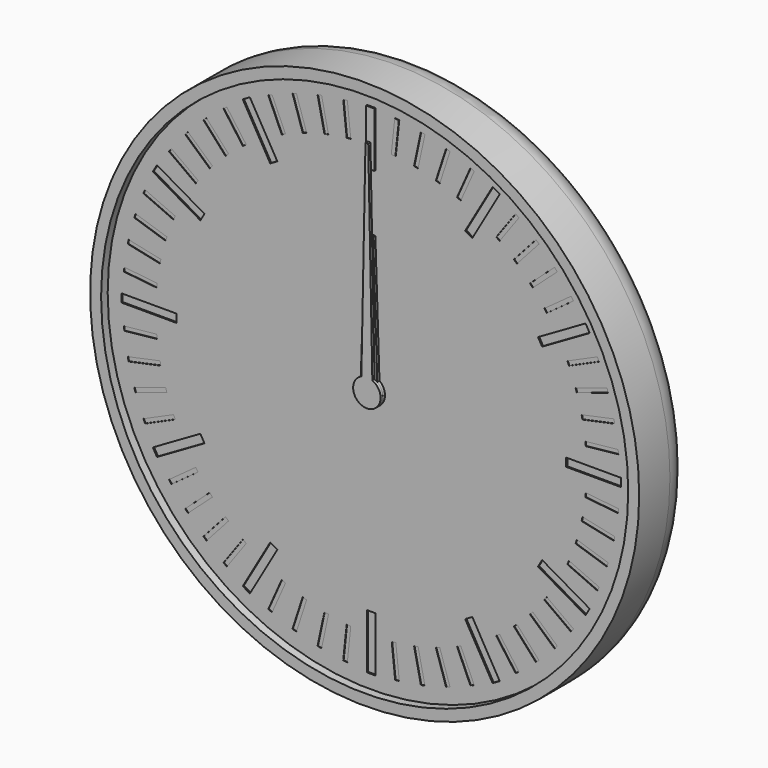
from build123d import *

# Parameters (mm, degrees)
F0_R      = 100
F1_DEPTH  = 24
F2_R      = 10
F3_T      = -4
F4_R      = 5
F4_R_2    = 3
F5_DEPTH  = 2
F6_DEPTH  = 19
F7_DEPTH  = 8
F9_DEPTH  = 4
F11_DEPTH = 4
F12_R     = 5
F12_R_2   = 3
F13_DEPTH = 2
F14_R     = 3
F15_DEPTH = 4
F17_DEPTH = 4
F18_R     = 3
F19_DEPTH = 4
F20_R     = 98
F20_R_2   = 5
F21_DEPTH = 1
F23_R     = 5
F23_R_2   = 3
F24_DEPTH = 4
F25_W     = 3
F25_H     = 20
F25_W_2   = 20
F25_H_2   = 3
F26_DEPTH = 0.5
F27_W     = 1.5
F27_H     = 12
F27_W_2   = 12
F27_H_2   = 1.5
F28_DEPTH = 0.2
F29_DEPTH = 1
F30_DEPTH = 0.4
F31_R     = 5
F31_R_2   = 3
F32_DEPTH = 5
F33_R     = 3
F34_DEPTH = 1
F36_DEPTH = 1


with BuildPart() as f1:
    # F0 (on Front) → F1 (new body)
    with BuildSketch(Plane.XZ):
        Circle(F0_R)
    extrude(amount=F1_DEPTH)

    # F2
    f2_edges = [f1.edges().sort_by_distance(p)[0] for p in [
        (-100, 0, 0),
    ]]
    fillet(f2_edges, radius=F2_R)

    # F3
    f3_openings = [f1.faces().sort_by_distance(p)[0] for p in [
        (0, -24, 0),
    ]]
    offset(amount=F3_T, openings=f3_openings)

    # F4 (on face) → F5 (join)
    with BuildSketch(Plane.XZ.offset(4)):
        Circle(F4_R)
        Circle(F4_R_2, mode=Mode.SUBTRACT)
        with Locations((40, 0)):
            Circle(F4_R)
        with Locations((40, 0)):
            Circle(F4_R_2, mode=Mode.SUBTRACT)
    extrude(amount=F5_DEPTH)


with BuildPart() as f6:
    # F6 (new): a face of the model
    f6_faces = [f1.part.faces().sort_by_distance(p)[0] for p in [
        (0, -4, 0),
    ]]
    extrude(f6_faces, amount=F6_DEPTH)

    # F8 (on face) → F9 (join)
    with BuildSketch(Plane.XZ.offset(6)):
        with BuildLine():
            ThreePointArc((9.2729637667, -1.3794085621), (9.3494561423, -0.6915886375), (9.375, 0))
            ThreePointArc((9.375, 0), (9.3494561423, 0.6915886375), (9.2729637667, 1.3794085621))
            ThreePointArc((9.2729637667, 1.3794085621), (8.9161548403, 2.8970343223), (8.3127812852, 4.3345463782))
            ThreePointArc((8.3127812852, 4.3345463782), (7.5845343223, 5.5104867402), (6.6911892658, 6.566476316))
            ThreePointArc((6.6911892658, 6.566476316), (5.5104867402, 7.5845343223), (4.1773988938, 8.3928519278))
            ThreePointArc((4.1773988938, 8.3928519278), (2.8970343223, 8.9161548403), (1.5536078905, 9.2453733036))
            ThreePointArc((1.5536078905, 9.2453733036), (0, 9.375), (-1.5536078905, 9.2453733036))
            ThreePointArc((-1.5536078905, 9.2453733036), (-2.8970343223, 8.9161548403), (-4.1773988938, 8.3928519278))
            ThreePointArc((-4.1773988938, 8.3928519278), (-5.5104867402, 7.5845343223), (-6.6911892658, 6.566476316))
            ThreePointArc((-6.6911892658, 6.566476316), (-7.5845343223, 5.5104867402), (-8.3127812852, 4.3345463782))
            ThreePointArc((-8.3127812852, 4.3345463782), (-8.9161548403, 2.8970343223), (-9.2729637667, 1.3794085621))
            ThreePointArc((-9.2729637667, 1.3794085621), (-9.375, 0), (-9.2729637667, -1.3794085621))
            ThreePointArc((-9.2729637667, -1.3794085621), (-8.9161548403, -2.8970343223), (-8.3127812852, -4.3345463782))
            ThreePointArc((-8.3127812852, -4.3345463782), (-7.5845343223, -5.5104867402), (-6.6911892658, -6.566476316))
            ThreePointArc((-6.6911892658, -6.566476316), (-5.5104867402, -7.5845343223), (-4.1773988938, -8.3928519278))
            ThreePointArc((-4.1773988938, -8.3928519278), (-2.8970343223, -8.9161548403), (-1.5536078905, -9.2453733036))
            ThreePointArc((-1.5536078905, -9.2453733036), (0, -9.375), (1.5536078905, -9.2453733036))
            ThreePointArc((1.5536078905, -9.2453733036), (2.8970343223, -8.9161548403), (4.1773988938, -8.3928519278))
            ThreePointArc((4.1773988938, -8.3928519278), (5.5104867402, -7.5845343223), (6.6911892658, -6.566476316))
            ThreePointArc((6.6911892658, -6.566476316), (7.5845343223, -5.5104867402), (8.3127812852, -4.3345463782))
            ThreePointArc((8.3127812852, -4.3345463782), (8.9161548403, -2.8970343223), (9.2729637667, -1.3794085621))
        make_face()
        with BuildLine():
            ThreePointArc((8.3127812852, 4.3345463782), (8.9161548403, 2.8970343223), (9.2729637667, 1.3794085621))
            Line((9.2729637667, 1.3794085621), (11.1823199426, 2.3946312492))
            Line((11.1823199426, 2.3946312492), (10.8182678729, 3.515068311))
            Line((10.8182678729, 3.515068311), (10.4542158031, 4.6355053728))
            Line((10.4542158031, 4.6355053728), (8.3127812852, 4.3345463782))
        make_face()
        with BuildLine():
            Line((11.1823199426, -2.3946312492), (9.2729637667, -1.3794085621))
            ThreePointArc((9.2729637667, -1.3794085621), (8.9161548403, -2.8970343223), (8.3127812852, -4.3345463782))
            Line((8.3127812852, -4.3345463782), (10.4542158031, -4.6355053728))
            Line((10.4542158031, -4.6355053728), (10.8182678729, -3.515068311))
            Line((10.8182678729, -3.515068311), (11.1823199426, -2.3946312492))
        make_face()
        with BuildLine():
            ThreePointArc((4.1773988938, 8.3928519278), (5.5104867402, 7.5845343223), (6.6911892658, 6.566476316))
            Line((6.6911892658, 6.566476316), (7.6391579371, 8.5101001246))
            Line((7.6391579371, 8.5101001246), (6.6860572448, 9.202568311))
            Line((6.6860572448, 9.202568311), (5.7329565525, 9.8950364974))
            Line((5.7329565525, 9.8950364974), (4.1773988938, 8.3928519278))
        make_face()
        with BuildLine():
            Line((7.6391579371, -8.5101001246), (6.6911892658, -6.566476316))
            ThreePointArc((6.6911892658, -6.566476316), (5.5104867402, -7.5845343223), (4.1773988938, -8.3928519278))
            Line((4.1773988938, -8.3928519278), (5.7329565525, -9.8950364974))
            Line((5.7329565525, -9.8950364974), (6.6860572448, -9.202568311))
            Line((6.6860572448, -9.202568311), (7.6391579371, -8.5101001246))
        make_face()
        with BuildLine():
            ThreePointArc((-1.5536078905, 9.2453733036), (0, 9.375), (1.5536078905, 9.2453733036))
            Line((1.5536078905, 9.2453733036), (1.1780972451, 11.375))
            Line((1.1780972451, 11.375), (0, 11.375))
            Line((0, 11.375), (-1.1780972451, 11.375))
            Line((-1.1780972451, 11.375), (-1.5536078905, 9.2453733036))
        make_face()
        with BuildLine():
            Line((1.1780972451, -11.375), (1.5536078905, -9.2453733036))
            ThreePointArc((1.5536078905, -9.2453733036), (0, -9.375), (-1.5536078905, -9.2453733036))
            Line((-1.5536078905, -9.2453733036), (-1.1780972451, -11.375))
            Line((-1.1780972451, -11.375), (0, -11.375))
            Line((0, -11.375), (1.1780972451, -11.375))
        make_face()
        with BuildLine():
            ThreePointArc((-6.6911892658, 6.566476316), (-5.5104867402, 7.5845343223), (-4.1773988938, 8.3928519278))
            Line((-4.1773988938, 8.3928519278), (-5.7329565525, 9.8950364974))
            Line((-5.7329565525, 9.8950364974), (-6.6860572448, 9.202568311))
            Line((-6.6860572448, 9.202568311), (-7.6391579371, 8.5101001246))
            Line((-7.6391579371, 8.5101001246), (-6.6911892658, 6.566476316))
        make_face()
        with BuildLine():
            Line((-5.7329565525, -9.8950364974), (-4.1773988938, -8.3928519278))
            ThreePointArc((-4.1773988938, -8.3928519278), (-5.5104867402, -7.5845343223), (-6.6911892658, -6.566476316))
            Line((-6.6911892658, -6.566476316), (-7.6391579371, -8.5101001246))
            Line((-7.6391579371, -8.5101001246), (-6.6860572448, -9.202568311))
            Line((-6.6860572448, -9.202568311), (-5.7329565525, -9.8950364974))
        make_face()
        with BuildLine():
            ThreePointArc((-9.2729637667, 1.3794085621), (-8.9161548403, 2.8970343223), (-8.3127812852, 4.3345463782))
            Line((-8.3127812852, 4.3345463782), (-10.4542158031, 4.6355053728))
            Line((-10.4542158031, 4.6355053728), (-10.8182678729, 3.515068311))
            Line((-10.8182678729, 3.515068311), (-11.1823199426, 2.3946312492))
            Line((-11.1823199426, 2.3946312492), (-9.2729637667, 1.3794085621))
        make_face()
        with BuildLine():
            Line((-10.4542158031, -4.6355053728), (-8.3127812852, -4.3345463782))
            ThreePointArc((-8.3127812852, -4.3345463782), (-8.9161548403, -2.8970343223), (-9.2729637667, -1.3794085621))
            Line((-9.2729637667, -1.3794085621), (-11.1823199426, -2.3946312492))
            Line((-11.1823199426, -2.3946312492), (-10.8182678729, -3.515068311))
            Line((-10.8182678729, -3.515068311), (-10.4542158031, -4.6355053728))
        make_face()
    extrude(amount=F9_DEPTH)

    # F35 (on face) → F36 (join)
    with BuildSketch(Plane.XZ.offset(23)):
        with BuildLine():
            ThreePointArc((-2, 4.582575695), (-2.7386127875, -4.1833001327), (5, 0))
            ThreePointArc((5, 0), (4.1833001327, 2.7386127875), (2, 4.582575695))
            ThreePointArc((2, 4.582575695), (0, 5), (-2, 4.582575695))
        make_face()
        with BuildLine():
            ThreePointArc((-2, 4.582575695), (0, 5), (2, 4.582575695))
            Line((2, 4.582575695), (0.5, 80))
            Line((0.5, 80), (0, 80))
            Line((0, 80), (-0.5, 80))
            Line((-0.5, 80), (-2, 4.582575695))
        make_face()
    extrude(amount=-F36_DEPTH)


with BuildPart() as f7:
    # F7 (new): a face of the model
    f7_faces = [f1.part.faces().sort_by_distance(p)[0] for p in [
        (40, -4, 0),
    ]]
    extrude(f7_faces, amount=F7_DEPTH)

    # F10 (on face) → F11 (join)
    with BuildSketch(Plane.XZ.offset(6)):
        with BuildLine():
            ThreePointArc((68.0829066802, -1.5381733945), (68.1144747006, -0.7693746225), (68.125, 0))
            ThreePointArc((68.125, 0), (68.1144747006, 0.7693746225), (68.0829066802, 1.5381733945))
            ThreePointArc((68.0829066802, 1.5381733945), (67.9709283072, 2.9398630294), (67.7890320221, 4.3342039956))
            ThreePointArc((67.7890320221, 4.3342039956), (67.5104012706, 5.8475163042), (67.1494235596, 7.3433252263))
            ThreePointArc((67.1494235596, 7.3433252263), (66.7484645208, 8.6911029668), (66.280643318, 10.0171558733))
            ThreePointArc((66.280643318, 10.0171558733), (65.6934659962, 11.4394680865), (65.0293803521, 12.8275385085))
            ThreePointArc((65.0293803521, 12.8275385085), (64.3569644814, 14.0625), (63.6236643925, 15.2623099717))
            ThreePointArc((63.6236643925, 15.2623099717), (62.7536029668, 16.5314602207), (61.815433119, 17.7511268046))
            ThreePointArc((61.815433119, 17.7511268046), (60.9009482166, 18.8192983038), (59.934217974, 19.8404278876))
            ThreePointArc((59.934217974, 19.8404278876), (58.8192983038, 20.9009482166), (57.6480467764, 21.8989056799))
            ThreePointArc((57.6480467764, 21.8989056799), (56.5314602207, 22.7536029668), (55.3735505752, 23.5514238999))
            ThreePointArc((55.3735505752, 23.5514238999), (54.0625, 24.3569644814), (52.709356105, 25.0895972944))
            ThreePointArc((52.709356105, 25.0895972944), (51.4394680865, 25.6934659962), (50.1409852457, 26.2331096755))
            ThreePointArc((50.1409852457, 26.2331096755), (48.6911029668, 26.7484645208), (47.2152055856, 27.1837531139))
            ThreePointArc((47.2152055856, 27.1837531139), (45.8475163042, 27.5104012706), (44.4652101991, 27.7682826779))
            ThreePointArc((44.4652101991, 27.7682826779), (42.9398630294, 27.9709283072), (41.4057159597, 28.0898484802))
            ThreePointArc((41.4057159597, 28.0898484802), (40, 28.125), (38.5942840403, 28.0898484802))
            ThreePointArc((38.5942840403, 28.0898484802), (37.0601369706, 27.9709283072), (35.5347898009, 27.7682826779))
            ThreePointArc((35.5347898009, 27.7682826779), (34.1524836958, 27.5104012706), (32.7847944144, 27.1837531139))
            ThreePointArc((32.7847944144, 27.1837531139), (31.3088970332, 26.7484645208), (29.8590147543, 26.2331096755))
            ThreePointArc((29.8590147543, 26.2331096755), (28.5605319135, 25.6934659962), (27.290643895, 25.0895972944))
            ThreePointArc((27.290643895, 25.0895972944), (25.9375, 24.3569644814), (24.6264494248, 23.5514238999))
            ThreePointArc((24.6264494248, 23.5514238999), (23.4685397793, 22.7536029668), (22.3519532236, 21.8989056799))
            ThreePointArc((22.3519532236, 21.8989056799), (21.1807016962, 20.9009482166), (20.065782026, 19.8404278876))
            ThreePointArc((20.065782026, 19.8404278876), (19.0990517834, 18.8192983038), (18.184566881, 17.7511268046))
            ThreePointArc((18.184566881, 17.7511268046), (17.2463970332, 16.5314602207), (16.3763356075, 15.2623099717))
            ThreePointArc((16.3763356075, 15.2623099717), (15.6430355186, 14.0625), (14.9706196479, 12.8275385085))
            ThreePointArc((14.9706196479, 12.8275385085), (14.3065340038, 11.4394680865), (13.719356682, 10.0171558733))
            ThreePointArc((13.719356682, 10.0171558733), (13.2515354792, 8.6911029668), (12.8505764404, 7.3433252263))
            ThreePointArc((12.8505764404, 7.3433252263), (12.4895987294, 5.8475163042), (12.2109679779, 4.3342039956))
            ThreePointArc((12.2109679779, 4.3342039956), (12.0290716928, 2.9398630294), (11.9170933198, 1.5381733945))
            ThreePointArc((11.9170933198, 1.5381733945), (11.875, 0), (11.9170933198, -1.5381733945))
            ThreePointArc((11.9170933198, -1.5381733945), (12.0290716928, -2.9398630294), (12.2109679779, -4.3342039956))
            ThreePointArc((12.2109679779, -4.3342039956), (12.4895987294, -5.8475163042), (12.8505764404, -7.3433252263))
            ThreePointArc((12.8505764404, -7.3433252263), (13.2515354792, -8.6911029668), (13.719356682, -10.0171558733))
            ThreePointArc((13.719356682, -10.0171558733), (14.3065340038, -11.4394680865), (14.9706196479, -12.8275385085))
            ThreePointArc((14.9706196479, -12.8275385085), (15.6430355186, -14.0625), (16.3763356075, -15.2623099717))
            ThreePointArc((16.3763356075, -15.2623099717), (17.2463970332, -16.5314602207), (18.184566881, -17.7511268046))
            ThreePointArc((18.184566881, -17.7511268046), (19.0990517834, -18.8192983038), (20.065782026, -19.8404278876))
            ThreePointArc((20.065782026, -19.8404278876), (21.1807016962, -20.9009482166), (22.3519532236, -21.8989056799))
            ThreePointArc((22.3519532236, -21.8989056799), (23.4685397793, -22.7536029668), (24.6264494248, -23.5514238999))
            ThreePointArc((24.6264494248, -23.5514238999), (25.9375, -24.3569644814), (27.290643895, -25.0895972944))
            ThreePointArc((27.290643895, -25.0895972944), (28.5605319135, -25.6934659962), (29.8590147543, -26.2331096755))
            ThreePointArc((29.8590147543, -26.2331096755), (31.3088970332, -26.7484645208), (32.7847944144, -27.1837531139))
            ThreePointArc((32.7847944144, -27.1837531139), (34.1524836958, -27.5104012706), (35.5347898009, -27.7682826779))
            ThreePointArc((35.5347898009, -27.7682826779), (37.0601369706, -27.9709283072), (38.5942840403, -28.0898484802))
            ThreePointArc((38.5942840403, -28.0898484802), (40, -28.125), (41.4057159597, -28.0898484802))
            ThreePointArc((41.4057159597, -28.0898484802), (42.9398630294, -27.9709283072), (44.4652101991, -27.7682826779))
            ThreePointArc((44.4652101991, -27.7682826779), (45.8475163042, -27.5104012706), (47.2152055856, -27.1837531139))
            ThreePointArc((47.2152055856, -27.1837531139), (48.6911029668, -26.7484645208), (50.1409852457, -26.2331096755))
            ThreePointArc((50.1409852457, -26.2331096755), (51.4394680865, -25.6934659962), (52.709356105, -25.0895972944))
            ThreePointArc((52.709356105, -25.0895972944), (54.0625, -24.3569644814), (55.3735505752, -23.5514238999))
            ThreePointArc((55.3735505752, -23.5514238999), (56.5314602207, -22.7536029668), (57.6480467764, -21.8989056799))
            ThreePointArc((57.6480467764, -21.8989056799), (58.8192983038, -20.9009482166), (59.934217974, -19.8404278876))
            ThreePointArc((59.934217974, -19.8404278876), (60.9009482166, -18.8192983038), (61.815433119, -17.7511268046))
            ThreePointArc((61.815433119, -17.7511268046), (62.7536029668, -16.5314602207), (63.6236643925, -15.2623099717))
            ThreePointArc((63.6236643925, -15.2623099717), (64.3569644814, -14.0625), (65.0293803521, -12.8275385085))
            ThreePointArc((65.0293803521, -12.8275385085), (65.6934659962, -11.4394680865), (66.280643318, -10.0171558733))
            ThreePointArc((66.280643318, -10.0171558733), (66.7484645208, -8.6911029668), (67.1494235596, -7.3433252263))
            ThreePointArc((67.1494235596, -7.3433252263), (67.5104012706, -5.8475163042), (67.7890320221, -4.3342039956))
            ThreePointArc((67.7890320221, -4.3342039956), (67.9709283072, -2.9398630294), (68.0829066802, -1.5381733945))
        make_face()
        with BuildLine():
            ThreePointArc((68.0829066802, 1.5381733945), (68.1144747006, 0.7693746225), (68.125, 0))
            ThreePointArc((68.125, 0), (68.1144747006, -0.7693746225), (68.0829066802, -1.5381733945))
            Line((68.0829066802, -1.5381733945), (70.125, -1.1780972451))
            Line((70.125, -1.1780972451), (70.125, 0))
            Line((70.125, 0), (70.125, 1.1780972451))
            Line((70.125, 1.1780972451), (68.0829066802, 1.5381733945))
        make_face()
        with BuildLine():
            ThreePointArc((67.1494235596, 7.3433252263), (67.5104012706, 5.8475163042), (67.7890320221, 4.3342039956))
            Line((67.7890320221, 4.3342039956), (69.7116366623, 5.1109866922))
            Line((69.7116366623, 5.1109866922), (69.4666964721, 6.2633396859))
            Line((69.4666964721, 6.2633396859), (69.2217562819, 7.4156926796))
            Line((69.2217562819, 7.4156926796), (67.1494235596, 7.3433252263))
        make_face()
        with BuildLine():
            Line((69.7116366623, -5.1109866922), (67.7890320221, -4.3342039956))
            ThreePointArc((67.7890320221, -4.3342039956), (67.5104012706, -5.8475163042), (67.1494235596, -7.3433252263))
            Line((67.1494235596, -7.3433252263), (69.2217562819, -7.4156926796))
            Line((69.2217562819, -7.4156926796), (69.4666964721, -6.2633396859))
            Line((69.4666964721, -6.2633396859), (69.7116366623, -5.1109866922))
        make_face()
        with BuildLine():
            ThreePointArc((65.0293803521, 12.8275385085), (65.6934659962, 11.4394680865), (66.280643318, 10.0171558733))
            Line((66.280643318, 10.0171558733), (67.9997322302, 11.1766959857))
            Line((67.9997322302, 11.1766959857), (67.5205569115, 12.2529413727))
            Line((67.5205569115, 12.2529413727), (67.0413815928, 13.3291867596))
            Line((67.0413815928, 13.3291867596), (65.0293803521, 12.8275385085))
        make_face()
        with BuildLine():
            Line((67.9997322302, -11.1766959857), (66.280643318, -10.0171558733))
            ThreePointArc((66.280643318, -10.0171558733), (65.6934659962, -11.4394680865), (65.0293803521, -12.8275385085))
            Line((65.0293803521, -12.8275385085), (67.0413815928, -13.3291867596))
            Line((67.0413815928, -13.3291867596), (67.5205569115, -12.2529413727))
            Line((67.5205569115, -12.2529413727), (67.9997322302, -11.1766959857))
        make_face()
        with BuildLine():
            ThreePointArc((61.815433119, 17.7511268046), (62.7536029668, 16.5314602207), (63.6236643925, 15.2623099717))
            Line((63.6236643925, 15.2623099717), (65.064105142, 16.753930033))
            Line((65.064105142, 16.753930033), (64.3716369555, 17.7070307253))
            Line((64.3716369555, 17.7070307253), (63.6791687691, 18.6601314176))
            Line((63.6791687691, 18.6601314176), (61.815433119, 17.7511268046))
        make_face()
        with BuildLine():
            Line((65.064105142, -16.753930033), (63.6236643925, -15.2623099717))
            ThreePointArc((63.6236643925, -15.2623099717), (62.7536029668, -16.5314602207), (61.815433119, -17.7511268046))
            Line((61.815433119, -17.7511268046), (63.6791687691, -18.6601314176))
            Line((63.6791687691, -18.6601314176), (64.3716369555, -17.7070307253))
            Line((64.3716369555, -17.7070307253), (65.064105142, -16.753930033))
        make_face()
        with BuildLine():
            ThreePointArc((57.6480467764, 21.8989056799), (58.8192983038, 20.9009482166), (59.934217974, 19.8404278876))
            Line((59.934217974, 19.8404278876), (61.0330563882, 21.5989369435))
            Line((61.0330563882, 21.5989369435), (60.1575595166, 22.3872378675))
            Line((60.1575595166, 22.3872378675), (59.282062645, 23.1755387915))
            Line((59.282062645, 23.1755387915), (57.6480467764, 21.8989056799))
        make_face()
        with BuildLine():
            Line((61.0330563882, -21.5989369435), (59.934217974, -19.8404278876))
            ThreePointArc((59.934217974, -19.8404278876), (58.8192983038, -20.9009482166), (57.6480467764, -21.8989056799))
            Line((57.6480467764, -21.8989056799), (59.282062645, -23.1755387915))
            Line((59.282062645, -23.1755387915), (60.1575595166, -22.3872378675))
            Line((60.1575595166, -22.3872378675), (61.0330563882, -21.5989369435))
        make_face()
        with BuildLine():
            ThreePointArc((52.709356105, 25.0895972944), (54.0625, 24.3569644814), (55.3735505752, 23.5514238999))
            Line((55.3735505752, 23.5514238999), (56.0827621424, 25.4999666665))
            Line((56.0827621424, 25.4999666665), (55.0625, 26.089015289))
            Line((55.0625, 26.089015289), (54.0422378576, 26.6780639116))
            Line((54.0422378576, 26.6780639116), (52.709356105, 25.0895972944))
        make_face()
        with BuildLine():
            Line((56.0827621424, -25.4999666665), (55.3735505752, -23.5514238999))
            ThreePointArc((55.3735505752, -23.5514238999), (54.0625, -24.3569644814), (52.709356105, -25.0895972944))
            Line((52.709356105, -25.0895972944), (54.0422378576, -26.6780639116))
            Line((54.0422378576, -26.6780639116), (55.0625, -26.089015289))
            Line((55.0625, -26.089015289), (56.0827621424, -25.4999666665))
        make_face()
        with BuildLine():
            ThreePointArc((47.2152055856, 27.1837531139), (48.6911029668, 26.7484645208), (50.1409852457, 26.2331096755))
            Line((50.1409852457, 26.2331096755), (50.4295740173, 28.2865254836))
            Line((50.4295740173, 28.2865254836), (49.3091369555, 28.6505775534))
            Line((49.3091369555, 28.6505775534), (48.1886998938, 29.0146296232))
            Line((48.1886998938, 29.0146296232), (47.2152055856, 27.1837531139))
        make_face()
        with BuildLine():
            Line((50.4295740173, -28.2865254836), (50.1409852457, -26.2331096755))
            ThreePointArc((50.1409852457, -26.2331096755), (48.6911029668, -26.7484645208), (47.2152055856, -27.1837531139))
            Line((47.2152055856, -27.1837531139), (48.1886998938, -29.0146296232))
            Line((48.1886998938, -29.0146296232), (49.3091369555, -28.6505775534))
            Line((49.3091369555, -28.6505775534), (50.4295740173, -28.2865254836))
        make_face()
        with BuildLine():
            ThreePointArc((41.4057159597, 28.0898484802), (42.9398630294, 27.9709283072), (44.4652101991, 27.7682826779))
            Line((44.4652101991, 27.7682826779), (44.3205634611, 29.8368274034))
            Line((44.3205634611, 29.8368274034), (43.1489199559, 29.959972098))
            Line((43.1489199559, 29.959972098), (41.9772764508, 30.0831167926))
            Line((41.9772764508, 30.0831167926), (41.4057159597, 28.0898484802))
        make_face()
        with BuildLine():
            Line((44.3205634611, -29.8368274034), (44.4652101991, -27.7682826779))
            ThreePointArc((44.4652101991, -27.7682826779), (42.9398630294, -27.9709283072), (41.4057159597, -28.0898484802))
            Line((41.4057159597, -28.0898484802), (41.9772764508, -30.0831167926))
            Line((41.9772764508, -30.0831167926), (43.1489199559, -29.959972098))
            Line((43.1489199559, -29.959972098), (44.3205634611, -29.8368274034))
        make_face()
        with BuildLine():
            ThreePointArc((35.5347898009, 27.7682826779), (37.0601369706, 27.9709283072), (38.5942840403, 28.0898484802))
            Line((38.5942840403, 28.0898484802), (38.0227235492, 30.0831167926))
            Line((38.0227235492, 30.0831167926), (36.8510800441, 29.959972098))
            Line((36.8510800441, 29.959972098), (35.6794365389, 29.8368274034))
            Line((35.6794365389, 29.8368274034), (35.5347898009, 27.7682826779))
        make_face()
        with BuildLine():
            Line((38.0227235492, -30.0831167926), (38.5942840403, -28.0898484802))
            ThreePointArc((38.5942840403, -28.0898484802), (37.0601369706, -27.9709283072), (35.5347898009, -27.7682826779))
            Line((35.5347898009, -27.7682826779), (35.6794365389, -29.8368274034))
            Line((35.6794365389, -29.8368274034), (36.8510800441, -29.959972098))
            Line((36.8510800441, -29.959972098), (38.0227235492, -30.0831167926))
        make_face()
        with BuildLine():
            ThreePointArc((29.8590147543, 26.2331096755), (31.3088970332, 26.7484645208), (32.7847944144, 27.1837531139))
            Line((32.7847944144, 27.1837531139), (31.8113001062, 29.0146296232))
            Line((31.8113001062, 29.0146296232), (30.6908630445, 28.6505775534))
            Line((30.6908630445, 28.6505775534), (29.5704259827, 28.2865254836))
            Line((29.5704259827, 28.2865254836), (29.8590147543, 26.2331096755))
        make_face()
        with BuildLine():
            Line((31.8113001062, -29.0146296232), (32.7847944144, -27.1837531139))
            ThreePointArc((32.7847944144, -27.1837531139), (31.3088970332, -26.7484645208), (29.8590147543, -26.2331096755))
            Line((29.8590147543, -26.2331096755), (29.5704259827, -28.2865254836))
            Line((29.5704259827, -28.2865254836), (30.6908630445, -28.6505775534))
            Line((30.6908630445, -28.6505775534), (31.8113001062, -29.0146296232))
        make_face()
        with BuildLine():
            ThreePointArc((24.6264494248, 23.5514238999), (25.9375, 24.3569644814), (27.290643895, 25.0895972944))
            Line((27.290643895, 25.0895972944), (25.9577621424, 26.6780639116))
            Line((25.9577621424, 26.6780639116), (24.9375, 26.089015289))
            Line((24.9375, 26.089015289), (23.9172378576, 25.4999666665))
            Line((23.9172378576, 25.4999666665), (24.6264494248, 23.5514238999))
        make_face()
        with BuildLine():
            Line((25.9577621424, -26.6780639116), (27.290643895, -25.0895972944))
            ThreePointArc((27.290643895, -25.0895972944), (25.9375, -24.3569644814), (24.6264494248, -23.5514238999))
            Line((24.6264494248, -23.5514238999), (23.9172378576, -25.4999666665))
            Line((23.9172378576, -25.4999666665), (24.9375, -26.089015289))
            Line((24.9375, -26.089015289), (25.9577621424, -26.6780639116))
        make_face()
        with BuildLine():
            ThreePointArc((20.065782026, 19.8404278876), (21.1807016962, 20.9009482166), (22.3519532236, 21.8989056799))
            Line((22.3519532236, 21.8989056799), (20.717937355, 23.1755387915))
            Line((20.717937355, 23.1755387915), (19.8424404834, 22.3872378675))
            Line((19.8424404834, 22.3872378675), (18.9669436118, 21.5989369435))
            Line((18.9669436118, 21.5989369435), (20.065782026, 19.8404278876))
        make_face()
        with BuildLine():
            Line((20.717937355, -23.1755387915), (22.3519532236, -21.8989056799))
            ThreePointArc((22.3519532236, -21.8989056799), (21.1807016962, -20.9009482166), (20.065782026, -19.8404278876))
            Line((20.065782026, -19.8404278876), (18.9669436118, -21.5989369435))
            Line((18.9669436118, -21.5989369435), (19.8424404834, -22.3872378675))
            Line((19.8424404834, -22.3872378675), (20.717937355, -23.1755387915))
        make_face()
        with BuildLine():
            ThreePointArc((16.3763356075, 15.2623099717), (17.2463970332, 16.5314602207), (18.184566881, 17.7511268046))
            Line((18.184566881, 17.7511268046), (16.3208312309, 18.6601314176))
            Line((16.3208312309, 18.6601314176), (15.6283630445, 17.7070307253))
            Line((15.6283630445, 17.7070307253), (14.935894858, 16.753930033))
            Line((14.935894858, 16.753930033), (16.3763356075, 15.2623099717))
        make_face()
        with BuildLine():
            Line((16.3208312309, -18.6601314176), (18.184566881, -17.7511268046))
            ThreePointArc((18.184566881, -17.7511268046), (17.2463970332, -16.5314602207), (16.3763356075, -15.2623099717))
            Line((16.3763356075, -15.2623099717), (14.935894858, -16.753930033))
            Line((14.935894858, -16.753930033), (15.6283630445, -17.7070307253))
            Line((15.6283630445, -17.7070307253), (16.3208312309, -18.6601314176))
        make_face()
        with BuildLine():
            ThreePointArc((13.719356682, 10.0171558733), (14.3065340038, 11.4394680865), (14.9706196479, 12.8275385085))
            Line((14.9706196479, 12.8275385085), (12.9586184072, 13.3291867596))
            Line((12.9586184072, 13.3291867596), (12.4794430885, 12.2529413727))
            Line((12.4794430885, 12.2529413727), (12.0002677698, 11.1766959857))
            Line((12.0002677698, 11.1766959857), (13.719356682, 10.0171558733))
        make_face()
        with BuildLine():
            Line((12.9586184072, -13.3291867596), (14.9706196479, -12.8275385085))
            ThreePointArc((14.9706196479, -12.8275385085), (14.3065340038, -11.4394680865), (13.719356682, -10.0171558733))
            Line((13.719356682, -10.0171558733), (12.0002677698, -11.1766959857))
            Line((12.0002677698, -11.1766959857), (12.4794430885, -12.2529413727))
            Line((12.4794430885, -12.2529413727), (12.9586184072, -13.3291867596))
        make_face()
        with BuildLine():
            ThreePointArc((12.2109679779, 4.3342039956), (12.4895987294, 5.8475163042), (12.8505764404, 7.3433252263))
            Line((12.8505764404, 7.3433252263), (10.7782437181, 7.4156926796))
            Line((10.7782437181, 7.4156926796), (10.5333035279, 6.2633396859))
            Line((10.5333035279, 6.2633396859), (10.2883633377, 5.1109866922))
            Line((10.2883633377, 5.1109866922), (12.2109679779, 4.3342039956))
        make_face()
        with BuildLine():
            Line((10.7782437181, -7.4156926796), (12.8505764404, -7.3433252263))
            ThreePointArc((12.8505764404, -7.3433252263), (12.4895987294, -5.8475163042), (12.2109679779, -4.3342039956))
            Line((12.2109679779, -4.3342039956), (10.2883633377, -5.1109866922))
            Line((10.2883633377, -5.1109866922), (10.5333035279, -6.2633396859))
            Line((10.5333035279, -6.2633396859), (10.7782437181, -7.4156926796))
        make_face()
        with BuildLine():
            ThreePointArc((11.9170933198, -1.5381733945), (11.875, 0), (11.9170933198, 1.5381733945))
            Line((11.9170933198, 1.5381733945), (9.875, 1.1780972451))
            Line((9.875, 1.1780972451), (9.875, 0))
            Line((9.875, 0), (9.875, -1.1780972451))
            Line((9.875, -1.1780972451), (11.9170933198, -1.5381733945))
        make_face()
    extrude(amount=F11_DEPTH)

    # F16 (on face) → F17 (join)
    with BuildSketch(Plane.XZ.offset(12)):
        with BuildLine():
            ThreePointArc((47.4288750323, -1.0304444454), (47.4821976298, -0.5164480894), (47.5, 0))
            ThreePointArc((47.5, 0), (47.4821976298, 0.5164480894), (47.4288750323, 1.0304444454))
            ThreePointArc((47.4288750323, 1.0304444454), (47.1329238722, 2.3176274578), (46.6157661985, 3.532936117))
            ThreePointArc((46.6157661985, 3.532936117), (46.0676274578, 4.4083893922), (45.4044061018, 5.2002302532))
            ThreePointArc((45.4044061018, 5.2002302532), (44.4083893922, 6.0676274578), (43.2756595386, 6.7468551628))
            ThreePointArc((43.2756595386, 6.7468551628), (42.3176274578, 7.1329238722), (41.3156377295, 7.3837048536))
            ThreePointArc((41.3156377295, 7.3837048536), (40, 7.5), (38.6843622705, 7.3837048536))
            ThreePointArc((38.6843622705, 7.3837048536), (37.6823725422, 7.1329238722), (36.7243404614, 6.7468551628))
            ThreePointArc((36.7243404614, 6.7468551628), (35.5916106078, 6.0676274578), (34.5955938982, 5.2002302532))
            ThreePointArc((34.5955938982, 5.2002302532), (33.9323725422, 4.4083893922), (33.3842338015, 3.532936117))
            ThreePointArc((33.3842338015, 3.532936117), (32.8670761278, 2.3176274578), (32.5711249677, 1.0304444454))
            ThreePointArc((32.5711249677, 1.0304444454), (32.5, 0), (32.5711249677, -1.0304444454))
            ThreePointArc((32.5711249677, -1.0304444454), (32.8670761278, -2.3176274578), (33.3842338015, -3.532936117))
            ThreePointArc((33.3842338015, -3.532936117), (33.9323725422, -4.4083893922), (34.5955938982, -5.2002302532))
            ThreePointArc((34.5955938982, -5.2002302532), (35.5916106078, -6.0676274578), (36.7243404614, -6.7468551628))
            ThreePointArc((36.7243404614, -6.7468551628), (37.6823725422, -7.1329238722), (38.6843622705, -7.3837048536))
            ThreePointArc((38.6843622705, -7.3837048536), (40, -7.5), (41.3156377295, -7.3837048536))
            ThreePointArc((41.3156377295, -7.3837048536), (42.3176274578, -7.1329238722), (43.2756595386, -6.7468551628))
            ThreePointArc((43.2756595386, -6.7468551628), (44.4083893922, -6.0676274578), (45.4044061018, -5.2002302532))
            ThreePointArc((45.4044061018, -5.2002302532), (46.0676274578, -4.4083893922), (46.6157661985, -3.532936117))
            ThreePointArc((46.6157661985, -3.532936117), (47.1329238722, -2.3176274578), (47.4288750323, -1.0304444454))
        make_face()
        with BuildLine():
            ThreePointArc((46.6157661985, 3.532936117), (47.1329238722, 2.3176274578), (47.4288750323, 1.0304444454))
            Line((47.4288750323, 1.0304444454), (49.3262785606, 2.0393117971))
            Line((49.3262785606, 2.0393117971), (48.743795249, 3.832011096))
            Line((48.743795249, 3.832011096), (46.6157661985, 3.532936117))
        make_face()
        with BuildLine():
            Line((49.3262785606, -2.0393117971), (47.4288750323, -1.0304444454))
            ThreePointArc((47.4288750323, -1.0304444454), (47.1329238722, -2.3176274578), (46.6157661985, -3.532936117))
            Line((46.6157661985, -3.532936117), (48.743795249, -3.832011096))
            Line((48.743795249, -3.832011096), (49.3262785606, -2.0393117971))
        make_face()
        with BuildLine():
            ThreePointArc((43.2756595386, 6.7468551628), (44.4083893922, 6.0676274578), (45.4044061018, 5.2002302532))
            Line((45.4044061018, 5.2002302532), (46.3464404506, 7.1316868974))
            Line((46.3464404506, 7.1316868974), (44.8214793429, 8.2396359957))
            Line((44.8214793429, 8.2396359957), (43.2756595386, 6.7468551628))
        make_face()
        with BuildLine():
            Line((46.3464404506, -7.1316868974), (45.4044061018, -5.2002302532))
            ThreePointArc((45.4044061018, -5.2002302532), (44.4083893922, -6.0676274578), (43.2756595386, -6.7468551628))
            Line((43.2756595386, -6.7468551628), (44.8214793429, -8.2396359957))
            Line((44.8214793429, -8.2396359957), (46.3464404506, -7.1316868974))
        make_face()
        with BuildLine():
            ThreePointArc((38.6843622705, 7.3837048536), (40, 7.5), (41.3156377295, 7.3837048536))
            Line((41.3156377295, 7.3837048536), (40.9424777961, 9.5))
            Line((40.9424777961, 9.5), (39.0575222039, 9.5))
            Line((39.0575222039, 9.5), (38.6843622705, 7.3837048536))
        make_face()
        with BuildLine():
            Line((40.9424777961, -9.5), (41.3156377295, -7.3837048536))
            ThreePointArc((41.3156377295, -7.3837048536), (40, -7.5), (38.6843622705, -7.3837048536))
            Line((38.6843622705, -7.3837048536), (39.0575222039, -9.5))
            Line((39.0575222039, -9.5), (40.9424777961, -9.5))
        make_face()
        with BuildLine():
            ThreePointArc((34.5955938982, 5.2002302532), (35.5916106078, 6.0676274578), (36.7243404614, 6.7468551628))
            Line((36.7243404614, 6.7468551628), (35.1785206571, 8.2396359957))
            Line((35.1785206571, 8.2396359957), (33.6535595494, 7.1316868974))
            Line((33.6535595494, 7.1316868974), (34.5955938982, 5.2002302532))
        make_face()
        with BuildLine():
            Line((35.1785206571, -8.2396359957), (36.7243404614, -6.7468551628))
            ThreePointArc((36.7243404614, -6.7468551628), (35.5916106078, -6.0676274578), (34.5955938982, -5.2002302532))
            Line((34.5955938982, -5.2002302532), (33.6535595494, -7.1316868974))
            Line((33.6535595494, -7.1316868974), (35.1785206571, -8.2396359957))
        make_face()
        with BuildLine():
            ThreePointArc((32.5711249677, 1.0304444454), (32.8670761278, 2.3176274578), (33.3842338015, 3.532936117))
            Line((33.3842338015, 3.532936117), (31.256204751, 3.832011096))
            Line((31.256204751, 3.832011096), (30.6737214394, 2.0393117971))
            Line((30.6737214394, 2.0393117971), (32.5711249677, 1.0304444454))
        make_face()
        with BuildLine():
            Line((31.256204751, -3.832011096), (33.3842338015, -3.532936117))
            ThreePointArc((33.3842338015, -3.532936117), (32.8670761278, -2.3176274578), (32.5711249677, -1.0304444454))
            Line((32.5711249677, -1.0304444454), (30.6737214394, -2.0393117971))
            Line((30.6737214394, -2.0393117971), (31.256204751, -3.832011096))
        make_face()
    extrude(amount=F17_DEPTH)

    # F18 (on face) → F19 (join)
    with BuildSketch(Plane.XZ.offset(16)):
        with Locations((40, 0)):
            Circle(F18_R)
    extrude(amount=F19_DEPTH)


with BuildPart() as f13:
    # F12 (on face) → F13 (new body)
    with BuildSketch(Plane.XZ.offset(10)):
        Circle(F12_R)
        Circle(F12_R_2, mode=Mode.SUBTRACT)
    extrude(amount=F13_DEPTH)

    # F14 (on face) → F15 (join)
    with BuildSketch(Plane.XZ.offset(12)):
        with BuildLine():
            ThreePointArc((29.9718156995, -1.3001014101), (29.9929530972, -0.6502034357), (30, 0))
            ThreePointArc((30, 0), (29.9929530972, 0.6502034357), (29.9718156995, 1.3001014101))
            ThreePointArc((29.9718156995, 1.3001014101), (29.907520012, 2.3537728718), (29.8061935814, 3.4045299509))
            ThreePointArc((29.8061935814, 3.4045299509), (29.6306502179, 4.6930339512), (29.3994322443, 5.9727199596))
            ThreePointArc((29.3994322443, 5.9727199596), (29.1710976119, 7.0033609157), (28.9066440563, 8.0253304855))
            ThreePointArc((28.9066440563, 8.0253304855), (28.5316954889, 9.2705098312), (28.1031371961, 10.4982703213))
            ThreePointArc((28.1031371961, 10.4982703213), (27.7163859753, 11.480502971), (27.2953170189, 12.448520749))
            ThreePointArc((27.2953170189, 12.448520749), (26.7301957257, 13.6197149922), (26.1148496411, 14.765318426))
            ThreePointArc((26.1148496411, 14.765318426), (25.5792049306, 15.6749569415), (25.0118886885, 16.5651871174))
            ThreePointArc((25.0118886885, 16.5651871174), (24.2705098312, 17.6335575688), (23.4835278178, 18.6687953878))
            ThreePointArc((23.4835278178, 18.6687953878), (22.812178968, 19.4834414499), (22.1125846489, 20.2739636023))
            ThreePointArc((22.1125846489, 20.2739636023), (21.2132034356, 21.2132034356), (20.2739636023, 22.1125846489))
            ThreePointArc((20.2739636023, 22.1125846489), (19.4834414499, 22.812178968), (18.6687953878, 23.4835278178))
            ThreePointArc((18.6687953878, 23.4835278178), (17.6335575688, 24.2705098312), (16.5651871174, 25.0118886885))
            ThreePointArc((16.5651871174, 25.0118886885), (15.6749569415, 25.5792049306), (14.765318426, 26.1148496411))
            ThreePointArc((14.765318426, 26.1148496411), (13.6197149922, 26.7301957257), (12.448520749, 27.2953170189))
            ThreePointArc((12.448520749, 27.2953170189), (11.480502971, 27.7163859753), (10.4982703213, 28.1031371961))
            ThreePointArc((10.4982703213, 28.1031371961), (9.2705098312, 28.5316954889), (8.0253304855, 28.9066440563))
            ThreePointArc((8.0253304855, 28.9066440563), (7.0033609157, 29.1710976119), (5.9727199596, 29.3994322443))
            ThreePointArc((5.9727199596, 29.3994322443), (4.6930339512, 29.6306502179), (3.4045299509, 29.8061935814))
            ThreePointArc((3.4045299509, 29.8061935814), (2.3537728718, 29.907520012), (1.3001014101, 29.9718156995))
            ThreePointArc((1.3001014101, 29.9718156995), (0, 30), (-1.3001014101, 29.9718156995))
            ThreePointArc((-1.3001014101, 29.9718156995), (-2.3537728718, 29.907520012), (-3.4045299509, 29.8061935814))
            ThreePointArc((-3.4045299509, 29.8061935814), (-4.6930339512, 29.6306502179), (-5.9727199596, 29.3994322443))
            ThreePointArc((-5.9727199596, 29.3994322443), (-7.0033609157, 29.1710976119), (-8.0253304855, 28.9066440563))
            ThreePointArc((-8.0253304855, 28.9066440563), (-9.2705098312, 28.5316954889), (-10.4982703213, 28.1031371961))
            ThreePointArc((-10.4982703213, 28.1031371961), (-11.480502971, 27.7163859753), (-12.448520749, 27.2953170189))
            ThreePointArc((-12.448520749, 27.2953170189), (-13.6197149922, 26.7301957257), (-14.765318426, 26.1148496411))
            ThreePointArc((-14.765318426, 26.1148496411), (-15.6749569415, 25.5792049306), (-16.5651871174, 25.0118886885))
            ThreePointArc((-16.5651871174, 25.0118886885), (-17.6335575688, 24.2705098312), (-18.6687953878, 23.4835278178))
            ThreePointArc((-18.6687953878, 23.4835278178), (-19.4834414499, 22.812178968), (-20.2739636023, 22.1125846489))
            ThreePointArc((-20.2739636023, 22.1125846489), (-21.2132034356, 21.2132034356), (-22.1125846489, 20.2739636023))
            ThreePointArc((-22.1125846489, 20.2739636023), (-22.812178968, 19.4834414499), (-23.4835278178, 18.6687953878))
            ThreePointArc((-23.4835278178, 18.6687953878), (-24.2705098312, 17.6335575688), (-25.0118886885, 16.5651871174))
            ThreePointArc((-25.0118886885, 16.5651871174), (-25.5792049306, 15.6749569415), (-26.1148496411, 14.765318426))
            ThreePointArc((-26.1148496411, 14.765318426), (-26.7301957257, 13.6197149922), (-27.2953170189, 12.448520749))
            ThreePointArc((-27.2953170189, 12.448520749), (-27.7163859753, 11.480502971), (-28.1031371961, 10.4982703213))
            ThreePointArc((-28.1031371961, 10.4982703213), (-28.5316954889, 9.2705098312), (-28.9066440563, 8.0253304855))
            ThreePointArc((-28.9066440563, 8.0253304855), (-29.1710976119, 7.0033609157), (-29.3994322443, 5.9727199596))
            ThreePointArc((-29.3994322443, 5.9727199596), (-29.6306502179, 4.6930339512), (-29.8061935814, 3.4045299509))
            ThreePointArc((-29.8061935814, 3.4045299509), (-29.907520012, 2.3537728718), (-29.9718156995, 1.3001014101))
            ThreePointArc((-29.9718156995, 1.3001014101), (-30, 0), (-29.9718156995, -1.3001014101))
            ThreePointArc((-29.9718156995, -1.3001014101), (-29.907520012, -2.3537728718), (-29.8061935814, -3.4045299509))
            ThreePointArc((-29.8061935814, -3.4045299509), (-29.6306502179, -4.6930339512), (-29.3994322443, -5.9727199596))
            ThreePointArc((-29.3994322443, -5.9727199596), (-29.1710976119, -7.0033609157), (-28.9066440563, -8.0253304855))
            ThreePointArc((-28.9066440563, -8.0253304855), (-28.5316954889, -9.2705098312), (-28.1031371961, -10.4982703213))
            ThreePointArc((-28.1031371961, -10.4982703213), (-27.7163859753, -11.480502971), (-27.2953170189, -12.448520749))
            ThreePointArc((-27.2953170189, -12.448520749), (-26.7301957257, -13.6197149922), (-26.1148496411, -14.765318426))
            ThreePointArc((-26.1148496411, -14.765318426), (-25.5792049306, -15.6749569415), (-25.0118886885, -16.5651871174))
            ThreePointArc((-25.0118886885, -16.5651871174), (-24.2705098312, -17.6335575688), (-23.4835278178, -18.6687953878))
            ThreePointArc((-23.4835278178, -18.6687953878), (-22.812178968, -19.4834414499), (-22.1125846489, -20.2739636023))
            ThreePointArc((-22.1125846489, -20.2739636023), (-21.2132034356, -21.2132034356), (-20.2739636023, -22.1125846489))
            ThreePointArc((-20.2739636023, -22.1125846489), (-19.4834414499, -22.812178968), (-18.6687953878, -23.4835278178))
            ThreePointArc((-18.6687953878, -23.4835278178), (-17.6335575688, -24.2705098312), (-16.5651871174, -25.0118886885))
            ThreePointArc((-16.5651871174, -25.0118886885), (-15.6749569415, -25.5792049306), (-14.765318426, -26.1148496411))
            ThreePointArc((-14.765318426, -26.1148496411), (-13.6197149922, -26.7301957257), (-12.448520749, -27.2953170189))
            ThreePointArc((-12.448520749, -27.2953170189), (-11.480502971, -27.7163859753), (-10.4982703213, -28.1031371961))
            ThreePointArc((-10.4982703213, -28.1031371961), (-9.2705098312, -28.5316954889), (-8.0253304855, -28.9066440563))
            ThreePointArc((-8.0253304855, -28.9066440563), (-7.0033609157, -29.1710976119), (-5.9727199596, -29.3994322443))
            ThreePointArc((-5.9727199596, -29.3994322443), (-4.6930339512, -29.6306502179), (-3.4045299509, -29.8061935814))
            ThreePointArc((-3.4045299509, -29.8061935814), (-2.3537728718, -29.907520012), (-1.3001014101, -29.9718156995))
            ThreePointArc((-1.3001014101, -29.9718156995), (0, -30), (1.3001014101, -29.9718156995))
            ThreePointArc((1.3001014101, -29.9718156995), (2.3537728718, -29.907520012), (3.4045299509, -29.8061935814))
            ThreePointArc((3.4045299509, -29.8061935814), (4.6930339512, -29.6306502179), (5.9727199596, -29.3994322443))
            ThreePointArc((5.9727199596, -29.3994322443), (7.0033609157, -29.1710976119), (8.0253304855, -28.9066440563))
            ThreePointArc((8.0253304855, -28.9066440563), (9.2705098312, -28.5316954889), (10.4982703213, -28.1031371961))
            ThreePointArc((10.4982703213, -28.1031371961), (11.480502971, -27.7163859753), (12.448520749, -27.2953170189))
            ThreePointArc((12.448520749, -27.2953170189), (13.6197149922, -26.7301957257), (14.765318426, -26.1148496411))
            ThreePointArc((14.765318426, -26.1148496411), (15.6749569415, -25.5792049306), (16.5651871174, -25.0118886885))
            ThreePointArc((16.5651871174, -25.0118886885), (17.6335575688, -24.2705098312), (18.6687953878, -23.4835278178))
            ThreePointArc((18.6687953878, -23.4835278178), (19.4834414499, -22.812178968), (20.2739636023, -22.1125846489))
            ThreePointArc((20.2739636023, -22.1125846489), (21.2132034356, -21.2132034356), (22.1125846489, -20.2739636023))
            ThreePointArc((22.1125846489, -20.2739636023), (22.812178968, -19.4834414499), (23.4835278178, -18.6687953878))
            ThreePointArc((23.4835278178, -18.6687953878), (24.2705098312, -17.6335575688), (25.0118886885, -16.5651871174))
            ThreePointArc((25.0118886885, -16.5651871174), (25.5792049306, -15.6749569415), (26.1148496411, -14.765318426))
            ThreePointArc((26.1148496411, -14.765318426), (26.7301957257, -13.6197149922), (27.2953170189, -12.448520749))
            ThreePointArc((27.2953170189, -12.448520749), (27.7163859753, -11.480502971), (28.1031371961, -10.4982703213))
            ThreePointArc((28.1031371961, -10.4982703213), (28.5316954889, -9.2705098312), (28.9066440563, -8.0253304855))
            ThreePointArc((28.9066440563, -8.0253304855), (29.1710976119, -7.0033609157), (29.3994322443, -5.9727199596))
            ThreePointArc((29.3994322443, -5.9727199596), (29.6306502179, -4.6930339512), (29.8061935814, -3.4045299509))
            ThreePointArc((29.8061935814, -3.4045299509), (29.907520012, -2.3537728718), (29.9718156995, -1.3001014101))
        make_face()
        Circle(F14_R, mode=Mode.SUBTRACT)
        with BuildLine():
            ThreePointArc((29.9718156995, 1.3001014101), (29.9929530972, 0.6502034357), (30, 0))
            ThreePointArc((30, 0), (29.9929530972, -0.6502034357), (29.9718156995, -1.3001014101))
            Line((29.9718156995, -1.3001014101), (32, -0.9424777961))
            Line((32, -0.9424777961), (32, 0))
            Line((32, 0), (32, 0.9424777961))
            Line((32, 0.9424777961), (29.9718156995, 1.3001014101))
        make_face()
        with BuildLine():
            ThreePointArc((29.3994322443, 5.9727199596), (29.6306502179, 4.6930339512), (29.8061935814, 3.4045299509))
            Line((29.8061935814, 3.4045299509), (31.7534629089, 4.0750285508))
            Line((31.7534629089, 4.0750285508), (31.606026899, 5.0059028813))
            Line((31.606026899, 5.0059028813), (31.4585908892, 5.9367772117))
            Line((31.4585908892, 5.9367772117), (29.3994322443, 5.9727199596))
        make_face()
        with BuildLine():
            Line((31.7534629089, -4.0750285508), (29.8061935814, -3.4045299509))
            ThreePointArc((29.8061935814, -3.4045299509), (29.6306502179, -4.6930339512), (29.3994322443, -5.9727199596))
            Line((29.3994322443, -5.9727199596), (31.4585908892, -5.9367772117))
            Line((31.4585908892, -5.9367772117), (31.606026899, -5.0059028813))
            Line((31.606026899, -5.0059028813), (31.7534629089, -4.0750285508))
        make_face()
        with BuildLine():
            ThreePointArc((28.1031371961, 10.4982703213), (28.5316954889, 9.2705098312), (28.9066440563, 8.0253304855))
            Line((28.9066440563, 8.0253304855), (30.7250501773, 8.9921941706))
            Line((30.7250501773, 8.9921941706), (30.4338085214, 9.88854382))
            Line((30.4338085214, 9.88854382), (30.1425668656, 10.7848934694))
            Line((30.1425668656, 10.7848934694), (28.1031371961, 10.4982703213))
        make_face()
        with BuildLine():
            Line((30.7250501773, -8.9921941706), (28.9066440563, -8.0253304855))
            ThreePointArc((28.9066440563, -8.0253304855), (28.5316954889, -9.2705098312), (28.1031371961, -10.4982703213))
            Line((28.1031371961, -10.4982703213), (30.1425668656, -10.7848934694))
            Line((30.1425668656, -10.7848934694), (30.4338085214, -9.88854382))
            Line((30.4338085214, -9.88854382), (30.7250501773, -8.9921941706))
        make_face()
        with BuildLine():
            ThreePointArc((26.1148496411, 14.765318426), (26.7301957257, 13.6197149922), (27.2953170189, 12.448520749))
            Line((27.2953170189, 12.448520749), (28.9400847397, 13.6879421265))
            Line((28.9400847397, 13.6879421265), (28.512208774, 14.5276959917))
            Line((28.512208774, 14.5276959917), (28.0843328084, 15.3674498569))
            Line((28.0843328084, 15.3674498569), (26.1148496411, 14.765318426))
        make_face()
        with BuildLine():
            Line((28.9400847397, -13.6879421265), (27.2953170189, -12.448520749))
            ThreePointArc((27.2953170189, -12.448520749), (26.7301957257, -13.6197149922), (26.1148496411, -14.765318426))
            Line((26.1148496411, -14.765318426), (28.0843328084, -15.3674498569))
            Line((28.0843328084, -15.3674498569), (28.512208774, -14.5276959917))
            Line((28.512208774, -14.5276959917), (28.9400847397, -13.6879421265))
        make_face()
        with BuildLine():
            ThreePointArc((23.4835278178, 18.6687953878), (24.2705098312, 17.6335575688), (25.0118886885, 16.5651871174))
            Line((25.0118886885, 16.5651871174), (26.4425183691, 18.0466475195))
            Line((26.4425183691, 18.0466475195), (25.88854382, 18.8091280734))
            Line((25.88854382, 18.8091280734), (25.3345692709, 19.5716086272))
            Line((25.3345692709, 19.5716086272), (23.4835278178, 18.6687953878))
        make_face()
        with BuildLine():
            Line((26.4425183691, -18.0466475195), (25.0118886885, -16.5651871174))
            ThreePointArc((25.0118886885, -16.5651871174), (24.2705098312, -17.6335575688), (23.4835278178, -18.6687953878))
            Line((23.4835278178, -18.6687953878), (25.3345692709, -19.5716086272))
            Line((25.3345692709, -19.5716086272), (25.88854382, -18.8091280734))
            Line((25.88854382, -18.8091280734), (26.4425183691, -18.0466475195))
        make_face()
        with BuildLine():
            ThreePointArc((20.2739636023, 22.1125846489), (21.2132034356, 21.2132034356), (22.1125846489, 20.2739636023))
            Line((22.1125846489, 20.2739636023), (23.2938494387, 21.9609845572))
            Line((23.2938494387, 21.9609845572), (22.627416998, 22.627416998))
            Line((22.627416998, 22.627416998), (21.9609845572, 23.2938494387))
            Line((21.9609845572, 23.2938494387), (20.2739636023, 22.1125846489))
        make_face()
        with BuildLine():
            Line((23.2938494387, -21.9609845572), (22.1125846489, -20.2739636023))
            ThreePointArc((22.1125846489, -20.2739636023), (21.2132034356, -21.2132034356), (20.2739636023, -22.1125846489))
            Line((20.2739636023, -22.1125846489), (21.9609845572, -23.2938494387))
            Line((21.9609845572, -23.2938494387), (22.627416998, -22.627416998))
            Line((22.627416998, -22.627416998), (23.2938494387, -21.9609845572))
        make_face()
        with BuildLine():
            ThreePointArc((16.5651871174, 25.0118886885), (17.6335575688, 24.2705098312), (18.6687953878, 23.4835278178))
            Line((18.6687953878, 23.4835278178), (19.5716086272, 25.3345692709))
            Line((19.5716086272, 25.3345692709), (18.8091280734, 25.88854382))
            Line((18.8091280734, 25.88854382), (18.0466475195, 26.4425183691))
            Line((18.0466475195, 26.4425183691), (16.5651871174, 25.0118886885))
        make_face()
        with BuildLine():
            Line((19.5716086272, -25.3345692709), (18.6687953878, -23.4835278178))
            ThreePointArc((18.6687953878, -23.4835278178), (17.6335575688, -24.2705098312), (16.5651871174, -25.0118886885))
            Line((16.5651871174, -25.0118886885), (18.0466475195, -26.4425183691))
            Line((18.0466475195, -26.4425183691), (18.8091280734, -25.88854382))
            Line((18.8091280734, -25.88854382), (19.5716086272, -25.3345692709))
        make_face()
        with BuildLine():
            ThreePointArc((12.448520749, 27.2953170189), (13.6197149922, 26.7301957257), (14.765318426, 26.1148496411))
            Line((14.765318426, 26.1148496411), (15.3674498569, 28.0843328084))
            Line((15.3674498569, 28.0843328084), (14.5276959917, 28.512208774))
            Line((14.5276959917, 28.512208774), (13.6879421265, 28.9400847397))
            Line((13.6879421265, 28.9400847397), (12.448520749, 27.2953170189))
        make_face()
        with BuildLine():
            Line((15.3674498569, -28.0843328084), (14.765318426, -26.1148496411))
            ThreePointArc((14.765318426, -26.1148496411), (13.6197149922, -26.7301957257), (12.448520749, -27.2953170189))
            Line((12.448520749, -27.2953170189), (13.6879421265, -28.9400847397))
            Line((13.6879421265, -28.9400847397), (14.5276959917, -28.512208774))
            Line((14.5276959917, -28.512208774), (15.3674498569, -28.0843328084))
        make_face()
        with BuildLine():
            ThreePointArc((8.0253304855, 28.9066440563), (9.2705098312, 28.5316954889), (10.4982703213, 28.1031371961))
            Line((10.4982703213, 28.1031371961), (10.7848934694, 30.1425668656))
            Line((10.7848934694, 30.1425668656), (9.88854382, 30.4338085214))
            Line((9.88854382, 30.4338085214), (8.9921941706, 30.7250501773))
            Line((8.9921941706, 30.7250501773), (8.0253304855, 28.9066440563))
        make_face()
        with BuildLine():
            Line((10.7848934694, -30.1425668656), (10.4982703213, -28.1031371961))
            ThreePointArc((10.4982703213, -28.1031371961), (9.2705098312, -28.5316954889), (8.0253304855, -28.9066440563))
            Line((8.0253304855, -28.9066440563), (8.9921941706, -30.7250501773))
            Line((8.9921941706, -30.7250501773), (9.88854382, -30.4338085214))
            Line((9.88854382, -30.4338085214), (10.7848934694, -30.1425668656))
        make_face()
        with BuildLine():
            ThreePointArc((3.4045299509, 29.8061935814), (4.6930339512, 29.6306502179), (5.9727199596, 29.3994322443))
            Line((5.9727199596, 29.3994322443), (5.9367772117, 31.4585908892))
            Line((5.9367772117, 31.4585908892), (5.0059028813, 31.606026899))
            Line((5.0059028813, 31.606026899), (4.0750285508, 31.7534629089))
            Line((4.0750285508, 31.7534629089), (3.4045299509, 29.8061935814))
        make_face()
        with BuildLine():
            Line((5.9367772117, -31.4585908892), (5.9727199596, -29.3994322443))
            ThreePointArc((5.9727199596, -29.3994322443), (4.6930339512, -29.6306502179), (3.4045299509, -29.8061935814))
            Line((3.4045299509, -29.8061935814), (4.0750285508, -31.7534629089))
            Line((4.0750285508, -31.7534629089), (5.0059028813, -31.606026899))
            Line((5.0059028813, -31.606026899), (5.9367772117, -31.4585908892))
        make_face()
        with BuildLine():
            ThreePointArc((-1.3001014101, 29.9718156995), (0, 30), (1.3001014101, 29.9718156995))
            Line((1.3001014101, 29.9718156995), (0.9424777961, 32))
            Line((0.9424777961, 32), (0, 32))
            Line((0, 32), (-0.9424777961, 32))
            Line((-0.9424777961, 32), (-1.3001014101, 29.9718156995))
        make_face()
        with BuildLine():
            Line((0.9424777961, -32), (1.3001014101, -29.9718156995))
            ThreePointArc((1.3001014101, -29.9718156995), (0, -30), (-1.3001014101, -29.9718156995))
            Line((-1.3001014101, -29.9718156995), (-0.9424777961, -32))
            Line((-0.9424777961, -32), (0, -32))
            Line((0, -32), (0.9424777961, -32))
        make_face()
        with BuildLine():
            ThreePointArc((-5.9727199596, 29.3994322443), (-4.6930339512, 29.6306502179), (-3.4045299509, 29.8061935814))
            Line((-3.4045299509, 29.8061935814), (-4.0750285508, 31.7534629089))
            Line((-4.0750285508, 31.7534629089), (-5.0059028813, 31.606026899))
            Line((-5.0059028813, 31.606026899), (-5.9367772117, 31.4585908892))
            Line((-5.9367772117, 31.4585908892), (-5.9727199596, 29.3994322443))
        make_face()
        with BuildLine():
            Line((-4.0750285508, -31.7534629089), (-3.4045299509, -29.8061935814))
            ThreePointArc((-3.4045299509, -29.8061935814), (-4.6930339512, -29.6306502179), (-5.9727199596, -29.3994322443))
            Line((-5.9727199596, -29.3994322443), (-5.9367772117, -31.4585908892))
            Line((-5.9367772117, -31.4585908892), (-5.0059028813, -31.606026899))
            Line((-5.0059028813, -31.606026899), (-4.0750285508, -31.7534629089))
        make_face()
        with BuildLine():
            ThreePointArc((-10.4982703213, 28.1031371961), (-9.2705098312, 28.5316954889), (-8.0253304855, 28.9066440563))
            Line((-8.0253304855, 28.9066440563), (-8.9921941706, 30.7250501773))
            Line((-8.9921941706, 30.7250501773), (-9.88854382, 30.4338085214))
            Line((-9.88854382, 30.4338085214), (-10.7848934694, 30.1425668656))
            Line((-10.7848934694, 30.1425668656), (-10.4982703213, 28.1031371961))
        make_face()
        with BuildLine():
            Line((-8.9921941706, -30.7250501773), (-8.0253304855, -28.9066440563))
            ThreePointArc((-8.0253304855, -28.9066440563), (-9.2705098312, -28.5316954889), (-10.4982703213, -28.1031371961))
            Line((-10.4982703213, -28.1031371961), (-10.7848934694, -30.1425668656))
            Line((-10.7848934694, -30.1425668656), (-9.88854382, -30.4338085214))
            Line((-9.88854382, -30.4338085214), (-8.9921941706, -30.7250501773))
        make_face()
        with BuildLine():
            ThreePointArc((-14.765318426, 26.1148496411), (-13.6197149922, 26.7301957257), (-12.448520749, 27.2953170189))
            Line((-12.448520749, 27.2953170189), (-13.6879421265, 28.9400847397))
            Line((-13.6879421265, 28.9400847397), (-14.5276959917, 28.512208774))
            Line((-14.5276959917, 28.512208774), (-15.3674498569, 28.0843328084))
            Line((-15.3674498569, 28.0843328084), (-14.765318426, 26.1148496411))
        make_face()
        with BuildLine():
            Line((-13.6879421265, -28.9400847397), (-12.448520749, -27.2953170189))
            ThreePointArc((-12.448520749, -27.2953170189), (-13.6197149922, -26.7301957257), (-14.765318426, -26.1148496411))
            Line((-14.765318426, -26.1148496411), (-15.3674498569, -28.0843328084))
            Line((-15.3674498569, -28.0843328084), (-14.5276959917, -28.512208774))
            Line((-14.5276959917, -28.512208774), (-13.6879421265, -28.9400847397))
        make_face()
        with BuildLine():
            ThreePointArc((-18.6687953878, 23.4835278178), (-17.6335575688, 24.2705098312), (-16.5651871174, 25.0118886885))
            Line((-16.5651871174, 25.0118886885), (-18.0466475195, 26.4425183691))
            Line((-18.0466475195, 26.4425183691), (-18.8091280734, 25.88854382))
            Line((-18.8091280734, 25.88854382), (-19.5716086272, 25.3345692709))
            Line((-19.5716086272, 25.3345692709), (-18.6687953878, 23.4835278178))
        make_face()
        with BuildLine():
            Line((-18.0466475195, -26.4425183691), (-16.5651871174, -25.0118886885))
            ThreePointArc((-16.5651871174, -25.0118886885), (-17.6335575688, -24.2705098312), (-18.6687953878, -23.4835278178))
            Line((-18.6687953878, -23.4835278178), (-19.5716086272, -25.3345692709))
            Line((-19.5716086272, -25.3345692709), (-18.8091280734, -25.88854382))
            Line((-18.8091280734, -25.88854382), (-18.0466475195, -26.4425183691))
        make_face()
        with BuildLine():
            ThreePointArc((-22.1125846489, 20.2739636023), (-21.2132034356, 21.2132034356), (-20.2739636023, 22.1125846489))
            Line((-20.2739636023, 22.1125846489), (-21.9609845572, 23.2938494387))
            Line((-21.9609845572, 23.2938494387), (-22.627416998, 22.627416998))
            Line((-22.627416998, 22.627416998), (-23.2938494387, 21.9609845572))
            Line((-23.2938494387, 21.9609845572), (-22.1125846489, 20.2739636023))
        make_face()
        with BuildLine():
            Line((-21.9609845572, -23.2938494387), (-20.2739636023, -22.1125846489))
            ThreePointArc((-20.2739636023, -22.1125846489), (-21.2132034356, -21.2132034356), (-22.1125846489, -20.2739636023))
            Line((-22.1125846489, -20.2739636023), (-23.2938494387, -21.9609845572))
            Line((-23.2938494387, -21.9609845572), (-22.627416998, -22.627416998))
            Line((-22.627416998, -22.627416998), (-21.9609845572, -23.2938494387))
        make_face()
        with BuildLine():
            ThreePointArc((-25.0118886885, 16.5651871174), (-24.2705098312, 17.6335575688), (-23.4835278178, 18.6687953878))
            Line((-23.4835278178, 18.6687953878), (-25.3345692709, 19.5716086272))
            Line((-25.3345692709, 19.5716086272), (-25.88854382, 18.8091280734))
            Line((-25.88854382, 18.8091280734), (-26.4425183691, 18.0466475195))
            Line((-26.4425183691, 18.0466475195), (-25.0118886885, 16.5651871174))
        make_face()
        with BuildLine():
            Line((-25.3345692709, -19.5716086272), (-23.4835278178, -18.6687953878))
            ThreePointArc((-23.4835278178, -18.6687953878), (-24.2705098312, -17.6335575688), (-25.0118886885, -16.5651871174))
            Line((-25.0118886885, -16.5651871174), (-26.4425183691, -18.0466475195))
            Line((-26.4425183691, -18.0466475195), (-25.88854382, -18.8091280734))
            Line((-25.88854382, -18.8091280734), (-25.3345692709, -19.5716086272))
        make_face()
        with BuildLine():
            ThreePointArc((-27.2953170189, 12.448520749), (-26.7301957257, 13.6197149922), (-26.1148496411, 14.765318426))
            Line((-26.1148496411, 14.765318426), (-28.0843328084, 15.3674498569))
            Line((-28.0843328084, 15.3674498569), (-28.512208774, 14.5276959917))
            Line((-28.512208774, 14.5276959917), (-28.9400847397, 13.6879421265))
            Line((-28.9400847397, 13.6879421265), (-27.2953170189, 12.448520749))
        make_face()
        with BuildLine():
            Line((-28.0843328084, -15.3674498569), (-26.1148496411, -14.765318426))
            ThreePointArc((-26.1148496411, -14.765318426), (-26.7301957257, -13.6197149922), (-27.2953170189, -12.448520749))
            Line((-27.2953170189, -12.448520749), (-28.9400847397, -13.6879421265))
            Line((-28.9400847397, -13.6879421265), (-28.512208774, -14.5276959917))
            Line((-28.512208774, -14.5276959917), (-28.0843328084, -15.3674498569))
        make_face()
        with BuildLine():
            ThreePointArc((-28.9066440563, 8.0253304855), (-28.5316954889, 9.2705098312), (-28.1031371961, 10.4982703213))
            Line((-28.1031371961, 10.4982703213), (-30.1425668656, 10.7848934694))
            Line((-30.1425668656, 10.7848934694), (-30.4338085214, 9.88854382))
            Line((-30.4338085214, 9.88854382), (-30.7250501773, 8.9921941706))
            Line((-30.7250501773, 8.9921941706), (-28.9066440563, 8.0253304855))
        make_face()
        with BuildLine():
            Line((-30.1425668656, -10.7848934694), (-28.1031371961, -10.4982703213))
            ThreePointArc((-28.1031371961, -10.4982703213), (-28.5316954889, -9.2705098312), (-28.9066440563, -8.0253304855))
            Line((-28.9066440563, -8.0253304855), (-30.7250501773, -8.9921941706))
            Line((-30.7250501773, -8.9921941706), (-30.4338085214, -9.88854382))
            Line((-30.4338085214, -9.88854382), (-30.1425668656, -10.7848934694))
        make_face()
        with BuildLine():
            ThreePointArc((-29.8061935814, 3.4045299509), (-29.6306502179, 4.6930339512), (-29.3994322443, 5.9727199596))
            Line((-29.3994322443, 5.9727199596), (-31.4585908892, 5.9367772117))
            Line((-31.4585908892, 5.9367772117), (-31.606026899, 5.0059028813))
            Line((-31.606026899, 5.0059028813), (-31.7534629089, 4.0750285508))
            Line((-31.7534629089, 4.0750285508), (-29.8061935814, 3.4045299509))
        make_face()
        with BuildLine():
            Line((-31.4585908892, -5.9367772117), (-29.3994322443, -5.9727199596))
            ThreePointArc((-29.3994322443, -5.9727199596), (-29.6306502179, -4.6930339512), (-29.8061935814, -3.4045299509))
            Line((-29.8061935814, -3.4045299509), (-31.7534629089, -4.0750285508))
            Line((-31.7534629089, -4.0750285508), (-31.606026899, -5.0059028813))
            Line((-31.606026899, -5.0059028813), (-31.4585908892, -5.9367772117))
        make_face()
        with BuildLine():
            ThreePointArc((-29.9718156995, -1.3001014101), (-30, 0), (-29.9718156995, 1.3001014101))
            Line((-29.9718156995, 1.3001014101), (-32, 0.9424777961))
            Line((-32, 0.9424777961), (-32, 0))
            Line((-32, 0), (-32, -0.9424777961))
            Line((-32, -0.9424777961), (-29.9718156995, -1.3001014101))
        make_face()
    extrude(amount=F15_DEPTH)

    # F31 (on face) → F32 (join)
    with BuildSketch(Plane.XZ.offset(16)):
        Circle(F31_R)
        Circle(F31_R_2, mode=Mode.SUBTRACT)
    extrude(amount=F32_DEPTH)

    # F33 (on face) → F34 (join)
    with BuildSketch(Plane.XZ.offset(21)):
        with BuildLine():
            ThreePointArc((-3, 4), (-2.2360679775, -4.472135955), (5, 0))
            ThreePointArc((5, 0), (4.472135955, 2.2360679775), (3, 4))
            ThreePointArc((3, 4), (0, 5), (-3, 4))
        make_face()
        Circle(F33_R, mode=Mode.SUBTRACT)
        with BuildLine():
            ThreePointArc((-3, 4), (0, 5), (3, 4))
            Line((3, 4), (1.5, 50))
            Line((1.5, 50), (0, 50))
            Line((0, 50), (-1.5, 50))
            Line((-1.5, 50), (-3, 4))
        make_face()
    extrude(amount=F34_DEPTH)


with BuildPart() as f21:
    # F20 (on face) → F21 (new body)
    with BuildSketch(Plane.XZ.offset(20)):
        Circle(F20_R)
        Circle(F20_R_2, mode=Mode.SUBTRACT)
    extrude(amount=F21_DEPTH)


with BuildPart() as f1_1:
    add(f1.part)

    # F22: cut F21
    add(f21.part, mode=Mode.SUBTRACT)


with BuildPart() as f21_1:
    add(f21.part)

    # F23 (on face) → F24 (join, through all)
    with BuildSketch(Plane(origin=(0, -20, 0), x_dir=(-1, 0, 0), z_dir=(0, 1, 0))):
        with Locations((-40, 0)):
            Circle(F23_R)
        with Locations((-40, 0)):
            Circle(F23_R_2, mode=Mode.SUBTRACT)
    extrude(amount=F24_DEPTH)

    # F25 (on face) → F26 (cut)
    with BuildSketch(Plane.XZ.offset(21)):
        with Locations((0, 81)):
            Rectangle(F25_W, F25_H)
        Polygon((-44.2009618943, 79.5583117444), (-46.7990381057, 78.0583117444), (-36.7990381057, 60.7378036687), (-34.2009618943, 62.2378036687), align=None)
        Polygon((-78.0583117444, 46.7990381057), (-79.5583117444, 44.2009618943), (-62.2378036687, 34.2009618943), (-60.7378036687, 36.7990381057), align=None)
        with Locations((-81, 0)):
            Rectangle(F25_W_2, F25_H_2)
        Polygon((-79.5583117444, -44.2009618943), (-78.0583117444, -46.7990381057), (-60.7378036687, -36.7990381057), (-62.2378036687, -34.2009618943), align=None)
        Polygon((-46.7990381057, -78.0583117444), (-44.2009618943, -79.5583117444), (-34.2009618943, -62.2378036687), (-36.7990381057, -60.7378036687), align=None)
        with Locations((0, -81)):
            Rectangle(F25_W, F25_H)
        Polygon((44.2009618943, -79.5583117444), (46.7990381057, -78.0583117444), (36.7990381057, -60.7378036687), (34.2009618943, -62.2378036687), align=None)
        Polygon((78.0583117444, -46.7990381057), (79.5583117444, -44.2009618943), (62.2378036687, -34.2009618943), (60.7378036687, -36.7990381057), align=None)
        with Locations((81, 0)):
            Rectangle(F25_W_2, F25_H_2)
        Polygon((79.5583117444, 44.2009618943), (78.0583117444, 46.7990381057), (60.7378036687, 36.7990381057), (62.2378036687, 34.2009618943), align=None)
        Polygon((46.7990381057, 78.0583117444), (44.2009618943, 79.5583117444), (34.2009618943, 62.2378036687), (36.7990381057, 60.7378036687), align=None)
    extrude(amount=-F26_DEPTH, mode=Mode.SUBTRACT)

    # F27 (on face) → F28 (cut)
    with BuildSketch(Plane.XZ.offset(21)):
        with Locations((0, 84.5)):
            Rectangle(F27_W, F27_H)
        Polygon((-8.7139345042, 90.0826278783), (-10.2057173472, 89.9258351834), (-8.951375788, 77.991572439), (-7.459592945, 78.1483651339), align=None)
        Polygon((-18.0823973185, 88.6782916345), (-19.5496187196, 88.3664240983), (-17.0546784297, 76.6286528895), (-15.5874570286, 76.9405204257), align=None)
        Polygon((-27.2527456037, 86.3023774705), (-28.6793303782, 85.8388519789), (-24.9711264457, 74.4261737834), (-23.5445416712, 74.889699275), align=None)
        Polygon((-36.1245071051, 82.980916399), (-37.4948252916, 82.3708114343), (-32.6139855747, 71.4082659426), (-31.2436673882, 72.0183709073), align=None)
        Polygon((-44.6004809472, 78.7502990425), (-45.8995190528, 78.0002990425), (-39.8995190528, 67.6079941971), (-38.6004809472, 68.3579941971), align=None)
        Polygon((-52.5878025867, 73.6568769302), (-53.8013280783, 72.7751990517), (-46.7479050507, 63.0669951192), (-45.5343795592, 63.9486729977), align=None)
        Polygon((-59.9989612564, 67.7564546605), (-61.1136784946, 66.7527587509), (-53.0841112183, 57.8350208452), (-51.9693939801, 58.8387167547), align=None)
        Polygon((-66.7527587509, 61.1136784946), (-67.7564546605, 59.9989612564), (-58.8387167547, 51.9693939801), (-57.8350208452, 53.0841112183), align=None)
        Polygon((-72.7751990517, 53.8013280783), (-73.6568769302, 52.5878025867), (-63.9486729977, 45.5343795592), (-63.0669951192, 46.7479050507), align=None)
        Polygon((-78.0002990425, 45.8995190528), (-78.7502990425, 44.6004809472), (-68.3579941971, 38.6004809472), (-67.6079941971, 39.8995190528), align=None)
        Polygon((-82.3708114343, 37.4948252916), (-82.980916399, 36.1245071051), (-72.0183709073, 31.2436673882), (-71.4082659426, 32.6139855747), align=None)
        Polygon((-85.8388519789, 28.6793303782), (-86.3023774705, 27.2527456037), (-74.889699275, 23.5445416712), (-74.4261737834, 24.9711264457), align=None)
        Polygon((-88.3664240983, 19.5496187196), (-88.6782916345, 18.0823973185), (-76.9405204257, 15.5874570286), (-76.6286528895, 17.0546784297), align=None)
        Polygon((-89.9258351834, 10.2057173472), (-90.0826278783, 8.7139345042), (-78.1483651339, 7.459592945), (-77.991572439, 8.951375788), align=None)
        with Locations((-84.5, 0)):
            Rectangle(F27_W_2, F27_H_2)
        Polygon((-90.0826278783, -8.7139345042), (-89.9258351834, -10.2057173472), (-77.991572439, -8.951375788), (-78.1483651339, -7.459592945), align=None)
        Polygon((-88.6782916345, -18.0823973185), (-88.3664240983, -19.5496187196), (-76.6286528895, -17.0546784297), (-76.9405204257, -15.5874570286), align=None)
        Polygon((-86.3023774705, -27.2527456037), (-85.8388519789, -28.6793303782), (-74.4261737834, -24.9711264457), (-74.889699275, -23.5445416712), align=None)
        Polygon((-82.980916399, -36.1245071051), (-82.3708114343, -37.4948252916), (-71.4082659426, -32.6139855747), (-72.0183709073, -31.2436673882), align=None)
        Polygon((-78.7502990425, -44.6004809472), (-78.0002990425, -45.8995190528), (-67.6079941971, -39.8995190528), (-68.3579941971, -38.6004809472), align=None)
        Polygon((-73.6568769302, -52.5878025867), (-72.7751990517, -53.8013280783), (-63.0669951192, -46.7479050507), (-63.9486729977, -45.5343795592), align=None)
        Polygon((-67.7564546605, -59.9989612564), (-66.7527587509, -61.1136784946), (-57.8350208452, -53.0841112183), (-58.8387167547, -51.9693939801), align=None)
        Polygon((-61.1136784946, -66.7527587509), (-59.9989612564, -67.7564546605), (-51.9693939801, -58.8387167547), (-53.0841112183, -57.8350208452), align=None)
        Polygon((-53.8013280783, -72.7751990517), (-52.5878025867, -73.6568769302), (-45.5343795592, -63.9486729977), (-46.7479050507, -63.0669951192), align=None)
        Polygon((-45.8995190528, -78.0002990425), (-44.6004809472, -78.7502990425), (-38.6004809472, -68.3579941971), (-39.8995190528, -67.6079941971), align=None)
        Polygon((-37.4948252916, -82.3708114343), (-36.1245071051, -82.980916399), (-31.2436673882, -72.0183709073), (-32.6139855747, -71.4082659426), align=None)
        Polygon((-28.6793303782, -85.8388519789), (-27.2527456037, -86.3023774705), (-23.5445416712, -74.889699275), (-24.9711264457, -74.4261737834), align=None)
        Polygon((-19.5496187196, -88.3664240983), (-18.0823973185, -88.6782916345), (-15.5874570286, -76.9405204257), (-17.0546784297, -76.6286528895), align=None)
        Polygon((-10.2057173472, -89.9258351834), (-8.7139345042, -90.0826278783), (-7.459592945, -78.1483651339), (-8.951375788, -77.991572439), align=None)
        with Locations((0, -84.5)):
            Rectangle(F27_W, F27_H)
        Polygon((8.7139345042, -90.0826278783), (10.2057173472, -89.9258351834), (8.951375788, -77.991572439), (7.459592945, -78.1483651339), align=None)
        Polygon((18.0823973185, -88.6782916345), (19.5496187196, -88.3664240983), (17.0546784297, -76.6286528895), (15.5874570286, -76.9405204257), align=None)
        Polygon((27.2527456037, -86.3023774705), (28.6793303782, -85.8388519789), (24.9711264457, -74.4261737834), (23.5445416712, -74.889699275), align=None)
        Polygon((36.1245071051, -82.980916399), (37.4948252916, -82.3708114343), (32.6139855747, -71.4082659426), (31.2436673882, -72.0183709073), align=None)
        Polygon((44.6004809472, -78.7502990425), (45.8995190528, -78.0002990425), (39.8995190528, -67.6079941971), (38.6004809472, -68.3579941971), align=None)
        Polygon((52.5878025867, -73.6568769302), (53.8013280783, -72.7751990517), (46.7479050507, -63.0669951192), (45.5343795592, -63.9486729977), align=None)
        Polygon((59.9989612564, -67.7564546605), (61.1136784946, -66.7527587509), (53.0841112183, -57.8350208452), (51.9693939801, -58.8387167547), align=None)
        Polygon((66.7527587509, -61.1136784946), (67.7564546605, -59.9989612564), (58.8387167547, -51.9693939801), (57.8350208452, -53.0841112183), align=None)
        Polygon((72.7751990517, -53.8013280783), (73.6568769302, -52.5878025867), (63.9486729977, -45.5343795592), (63.0669951192, -46.7479050507), align=None)
        Polygon((78.0002990425, -45.8995190528), (78.7502990425, -44.6004809472), (68.3579941971, -38.6004809472), (67.6079941971, -39.8995190528), align=None)
        Polygon((82.3708114343, -37.4948252916), (82.980916399, -36.1245071051), (72.0183709073, -31.2436673882), (71.4082659426, -32.6139855747), align=None)
        Polygon((85.8388519789, -28.6793303782), (86.3023774705, -27.2527456037), (74.889699275, -23.5445416712), (74.4261737834, -24.9711264457), align=None)
        Polygon((88.3664240983, -19.5496187196), (88.6782916345, -18.0823973185), (76.9405204257, -15.5874570286), (76.6286528895, -17.0546784297), align=None)
        Polygon((89.9258351834, -10.2057173472), (90.0826278783, -8.7139345042), (78.1483651339, -7.459592945), (77.991572439, -8.951375788), align=None)
        with Locations((84.5, 0)):
            Rectangle(F27_W_2, F27_H_2)
        Polygon((90.0826278783, 8.7139345042), (89.9258351834, 10.2057173472), (77.991572439, 8.951375788), (78.1483651339, 7.459592945), align=None)
        Polygon((88.6782916345, 18.0823973185), (88.3664240983, 19.5496187196), (76.6286528895, 17.0546784297), (76.9405204257, 15.5874570286), align=None)
        Polygon((86.3023774705, 27.2527456037), (85.8388519789, 28.6793303782), (74.4261737834, 24.9711264457), (74.889699275, 23.5445416712), align=None)
        Polygon((82.980916399, 36.1245071051), (82.3708114343, 37.4948252916), (71.4082659426, 32.6139855747), (72.0183709073, 31.2436673882), align=None)
        Polygon((78.7502990425, 44.6004809472), (78.0002990425, 45.8995190528), (67.6079941971, 39.8995190528), (68.3579941971, 38.6004809472), align=None)
        Polygon((73.6568769302, 52.5878025867), (72.7751990517, 53.8013280783), (63.0669951192, 46.7479050507), (63.9486729977, 45.5343795592), align=None)
        Polygon((67.7564546605, 59.9989612564), (66.7527587509, 61.1136784946), (57.8350208452, 53.0841112183), (58.8387167547, 51.9693939801), align=None)
        Polygon((61.1136784946, 66.7527587509), (59.9989612564, 67.7564546605), (51.9693939801, 58.8387167547), (53.0841112183, 57.8350208452), align=None)
        Polygon((53.8013280783, 72.7751990517), (52.5878025867, 73.6568769302), (45.5343795592, 63.9486729977), (46.7479050507, 63.0669951192), align=None)
        Polygon((45.8995190528, 78.0002990425), (44.6004809472, 78.7502990425), (38.6004809472, 68.3579941971), (39.8995190528, 67.6079941971), align=None)
        Polygon((37.4948252916, 82.3708114343), (36.1245071051, 82.980916399), (31.2436673882, 72.0183709073), (32.6139855747, 71.4082659426), align=None)
        Polygon((28.6793303782, 85.8388519789), (27.2527456037, 86.3023774705), (23.5445416712, 74.889699275), (24.9711264457, 74.4261737834), align=None)
        Polygon((19.5496187196, 88.3664240983), (18.0823973185, 88.6782916345), (15.5874570286, 76.9405204257), (17.0546784297, 76.6286528895), align=None)
        Polygon((10.2057173472, 89.9258351834), (8.7139345042, 90.0826278783), (7.459592945, 78.1483651339), (8.951375788, 77.991572439), align=None)
    extrude(amount=-F28_DEPTH, mode=Mode.SUBTRACT)


with BuildPart() as f29:
    # F29 (new): a face of the model
    f29_faces = [f21_1.part.faces().sort_by_distance(p)[0] for p in [
        (0, -20.5, 81),
    ]]
    extrude(f29_faces, amount=F29_DEPTH)


with BuildPart() as f30:
    # F30 (new): a face of the model
    f30_faces = [f21_1.part.faces().sort_by_distance(p)[0] for p in [
        (8.8326551461, -20.8, 84.0371001586),
    ]]
    extrude(f30_faces, amount=F30_DEPTH)


solid = Compound([f6.part, f7.part, f13.part, f1_1.part, f21_1.part, f29.part, f30.part])
